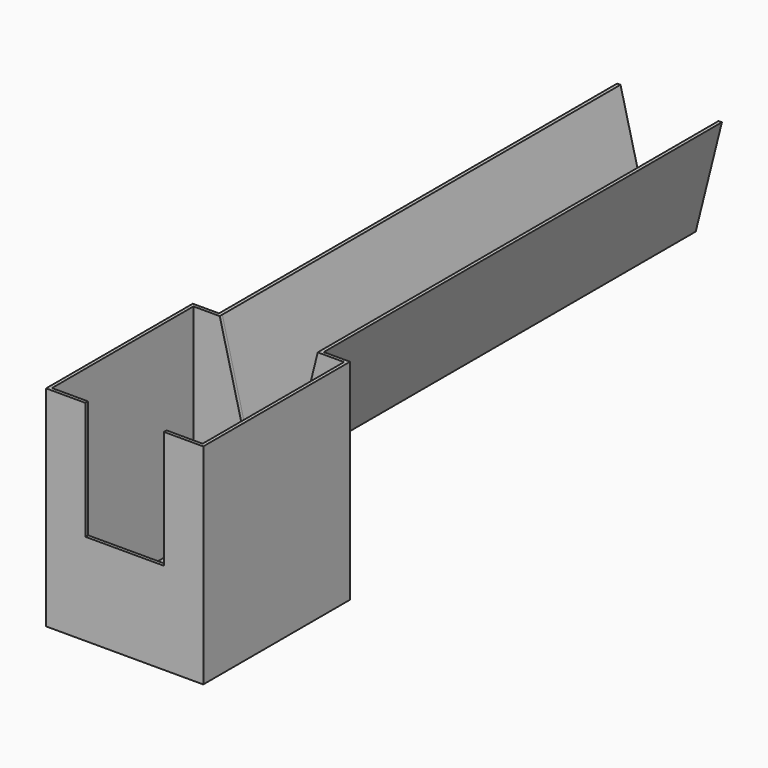
from build123d import *

# Parameters (mm, degrees)
F1_DEPTH    = 508
F3_DEPTH    = 177.8
F4_T        = 3.175
F4_T3_DEPTH = 111.0768828907
F4_T5_DEPTH = 57.15
F4_T7_DEPTH = 111.0768828907
F6_DEPTH    = 25.4
F8_DEPTH    = 25.4


# Not quite as in the source:
# - a shell that OpenCascade refuses in one call is made with other operations: the cavity is built on its own and cut out


with BuildPart() as f1:
    # F0 (on Front) → F1 (new body)
    with BuildSketch(Plane.XZ):
        Polygon((-25.4, 0), (0, 0), (25.4, 0), (50.8, 101.6), (-50.8, 101.6), align=None)
    extrude(amount=-F1_DEPTH)

    # F2 (on Front) → F3 (join)
    with BuildSketch(Plane.XZ):
        Polygon((76.2, -101.6), (76.2, 0), (76.2, 101.6), (-76.2, 101.6), (-76.2, 0), (-76.2, -101.6), align=None)
    extrude(amount=F3_DEPTH)

    # F4: shell of thickness 3.175, made by hand


with BuildPart() as f4_core1:
    # F4_t2: copy of F1
    add(f1.part)

    # the walls: a layer under each face that stays
    f4_faces = [f4_core1.faces().sort_by_distance(p)[0] for p in [
        (76.2, -88.9, 0),
        (0, -88.9, -101.6),
        (0, -177.8, 0),
        (-50.8, 0, -67.7333333333),
        (-76.2, -88.9, 0),
        (-38.1, 254, 50.8),
        (0, 254, 0),
        (38.1, 254, 50.8),
        (0, 508, 50.8),
    ]]
    thicken(f4_faces, amount=-F4_T, mode=Mode.SUBTRACT)

    # F4_s4 → F4_t3 (cut)
    with BuildSketch(Plane(origin=(-27.6641682565, 0, 110.6566730262), x_dir=(0, 1, 0), z_dir=(0.242535625, 0, -0.9701425001))):
        Polygon((0.03175, -24.6733695037), (-3.175, -24.6416195037), (-3.175, -21.4666195037), (0, -21.4666195037), align=None)
    extrude(amount=F4_T3_DEPTH, mode=Mode.SUBTRACT)

    # F4_s6 → F4_t5 (cut)
    with BuildSketch(Plane.YZ.offset(-28.575)):
        Polygon((0.03175, -0.03175), (-3.175, 0), (-3.175, 3.175), (0, 3.175), align=None)
    extrude(amount=F4_T5_DEPTH, mode=Mode.SUBTRACT)

    # F4_s8 → F4_t7 (cut)
    with BuildSketch(Plane(origin=(0.7240670376, 0, 2.8962681503), x_dir=(0, 1, 0), z_dir=(0.242535625, 0, 0.9701425001))):
        Polygon((0.03175, -24.6733695037), (-3.175, -24.6416195037), (-3.175, -21.4666195037), (0, -21.4666195037), align=None)
    extrude(amount=F4_T7_DEPTH, mode=Mode.SUBTRACT)


with BuildPart() as f1_1:
    add(f1.part)

    # what is left inside the walls is the cavity
    f4_cavity = [f4_core1.part.solids().sort_by_distance(p)[0] for p in [
        (0, 51.858333, 101.56825),
    ]]
    add(f4_cavity, mode=Mode.SUBTRACT)

    # F5 (on face) → F6 (cut)
    with BuildSketch(Plane(origin=(0, 508, 0), x_dir=(-1, 0, 0), z_dir=(0, 1, 0))):
        Polygon((-47.5272849097, 101.6), (-50.8, 101.6), (-50.00625, 98.425), (-25.4, 0), (25.4, 0), (50.00625, 98.425), (50.8, 101.6), (47.5272849097, 101.6), (46.7335349097, 98.425), (22.9210349097, 3.175), (-22.9210349097, 3.175), (-46.7335349097, 98.425), align=None)
        Polygon((47.5272849097, 101.6), (-47.5272849097, 101.6), (-46.7335349097, 98.425), (-22.9210349097, 3.175), (22.9210349097, 3.175), (46.7335349097, 98.425), align=None)
    extrude(amount=-F6_DEPTH, mode=Mode.SUBTRACT)

    # F7 (on face) → F8 (cut)
    with BuildSketch(Plane.XZ.offset(177.8)):
        Polygon((-38.1, -12.7), (0, -12.7), (38.1, -12.7), (38.1, 101.6), (-38.1, 101.6), align=None)
    extrude(amount=-F8_DEPTH, mode=Mode.SUBTRACT)


solid = f1_1.part
